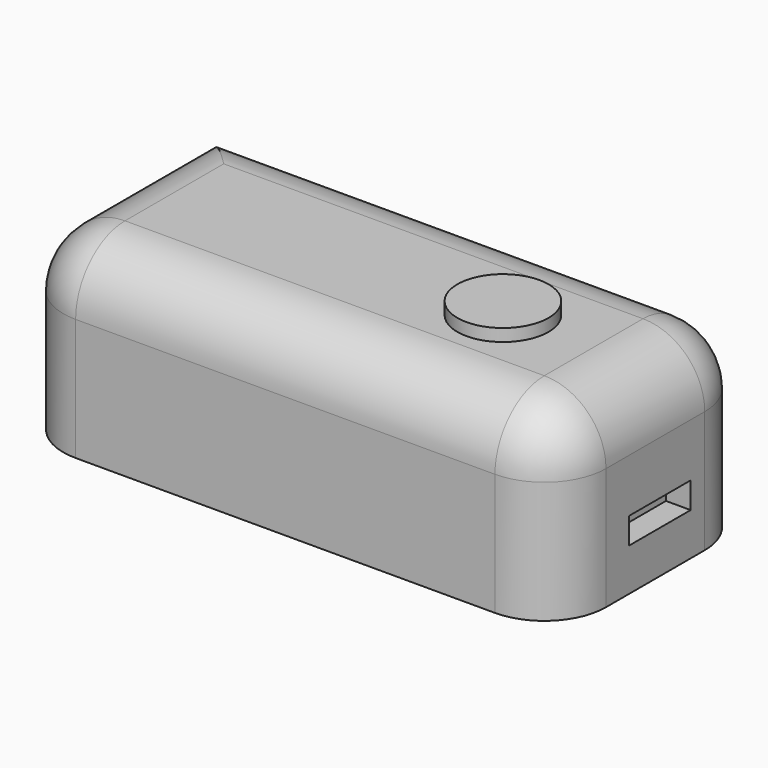
from build123d import *

# Parameters (mm, degrees)
F0_W         = 111.723061651
F0_H         = 37.8229115158
F1_DEPTH     = 50.8
F2_R         = 12.7
F3_T1_DEPTH  = 56.8729115158
F3_S5_W      = 12.7
F3_S5_H      = 12.7
F3_T6_DEPTH  = 12.7
F3_S11_W     = 12.7
F3_S11_H     = 12.7
F3_T12_DEPTH = 12.7
F3_S17_W     = 12.7
F3_S17_H     = 12.7
F3_T18_DEPTH = 12.7
F4_W         = 15.8335566521
F4_H         = 5.3901481442
F5_DEPTH     = 5.08
F6_R         = 9.3845015794
F7_DEPTH     = 2.54


# Not quite as in the source:
# - a fillet or chamfer that OpenCascade refuses, or shapes differently, is made with other operations: its cross-section is extruded or revolved along the edge and cut away or added


with BuildPart() as f1:
    # F0 (on Front) → F1 (new body)
    with BuildSketch(Plane.XZ):
        with Locations((3.3458750695, -1.4644479379)):
            Rectangle(F0_W, F0_H)
    extrude(amount=F1_DEPTH)

    # F2
    f2_edges = [f1.edges().sort_by_distance(p)[0] for p in [
        (59.207406, -25.4, 17.447008),
        (-52.515656, -25.4, 17.447008),
        (3.345875, 0, 17.447008),
        (3.345875, -50.8, 17.447008),
    ]]
    fillet(f2_edges, radius=F2_R)

    # F3: fillet of radius 12.7 on 7 edges, made by hand

    # F3_s2 → F3_t1 (cut)
    with BuildSketch(Plane.XY.offset(-52.1259036958)):
        with BuildLine():
            ThreePointArc((-39.815655756, -50.8), (-48.7959118771, -47.0802561211), (-52.515655756, -38.1))
            Line((-52.515655756, -38.1), (-52.515655756, -50.8))
            Line((-52.515655756, -50.8), (-39.815655756, -50.8))
        make_face()
        with BuildLine():
            ThreePointArc((59.207405895, -38.1), (55.4876620161, -47.0802561211), (46.507405895, -50.8))
            Line((46.507405895, -50.8), (59.207405895, -50.8))
            Line((59.207405895, -50.8), (59.207405895, -38.1))
        make_face()
        with BuildLine():
            ThreePointArc((59.207405895, -12.7), (55.4876620161, -3.7197438789), (46.507405895, 0))
            Line((46.507405895, 0), (59.207405895, 0))
            Line((59.207405895, 0), (59.207405895, -12.7))
        make_face()
    extrude(amount=F3_T1_DEPTH, mode=Mode.SUBTRACT)


with BuildPart() as f3_tool4:
    # F3_s5 → F3_t6 (new body)
    with BuildSketch(Plane.YZ.offset(46.507405895)):
        with Locations((-6.35, 11.09700782)):
            Rectangle(F3_S5_W, F3_S5_H)
    extrude(amount=F3_T6_DEPTH)

    # F3_s7 → F3_t8 (revolve, cut)
    with BuildSketch(Plane(origin=(46.507405895, -12.7, 4.74700782), x_dir=(0, -0.7071067812, -0.7071067812), z_dir=(0, -0.7071067812, 0.7071067812))):
        with BuildLine():
            ThreePointArc((0, -12.7), (12.7, 0), (0, 12.7))
            Line((0, 12.7), (0, -12.7))
        make_face()
    revolve(axis=Axis((46.507405895, -12.7, 4.74700782), (1, 0, 0)), mode=Mode.SUBTRACT)


with BuildPart() as f1_1:
    add(f1.part)

    # F3_t3: cut F3_tool4
    add(f3_tool4.part, mode=Mode.SUBTRACT)


with BuildPart() as f3_tool10:
    # F3_s11 → F3_t12 (new body)
    with BuildSketch(Plane.YZ.offset(46.507405895)):
        with Locations((-44.45, 11.09700782)):
            Rectangle(F3_S11_W, F3_S11_H)
    extrude(amount=F3_T12_DEPTH)

    # F3_s13 → F3_t14 (revolve, cut)
    with BuildSketch(Plane(origin=(46.507405895, -38.1, 4.74700782), x_dir=(0, 0.7071067812, -0.7071067812), z_dir=(0, -0.7071067812, -0.7071067812))):
        with BuildLine():
            ThreePointArc((0, -12.7), (12.7, 0), (0, 12.7))
            Line((0, 12.7), (0, -12.7))
        make_face()
    revolve(axis=Axis((46.507405895, -38.1, 4.74700782), (1, 0, 0)), mode=Mode.SUBTRACT)


with BuildPart() as f1_2:
    add(f1_1.part)

    # F3_t9: cut F3_tool10
    add(f3_tool10.part, mode=Mode.SUBTRACT)


with BuildPart() as f3_tool16:
    # F3_s17 → F3_t18 (new body)
    with BuildSketch(Plane.XZ.offset(38.1)):
        with Locations((-46.165655756, 11.09700782)):
            Rectangle(F3_S17_W, F3_S17_H)
    extrude(amount=F3_T18_DEPTH)

    # F3_s19 → F3_t20 (revolve, cut)
    with BuildSketch(Plane(origin=(-39.815655756, -38.1, 4.74700782), x_dir=(0.7071067812, 0, -0.7071067812), z_dir=(-0.7071067812, 0, -0.7071067812))):
        with BuildLine():
            ThreePointArc((0, -12.7), (12.7, 0), (0, 12.7))
            Line((0, 12.7), (0, -12.7))
        make_face()
    revolve(axis=Axis((-39.815655756, -38.1, 4.74700782), (0, -1, 0)), mode=Mode.SUBTRACT)


with BuildPart() as f1_3:
    add(f1_2.part)

    # F3_t15: cut F3_tool16
    add(f3_tool16.part, mode=Mode.SUBTRACT)

    # F4 (on face) → F5 (cut)
    with BuildSketch(Plane.YZ.offset(59.207405895)):
        with Locations((-24.2352448404, -8.9274321217)):
            Rectangle(F4_W, F4_H)
    extrude(amount=-F5_DEPTH, mode=Mode.SUBTRACT)


with BuildPart() as f7:
    # F6 (on face) → F7 (new body)
    with BuildSketch(Plane.XY.offset(17.44700782)):
        with Locations((28.1298365444, -25.7716421038)):
            Circle(F6_R)
    extrude(amount=F7_DEPTH)


solid = Compound([f1_3.part, f7.part])
